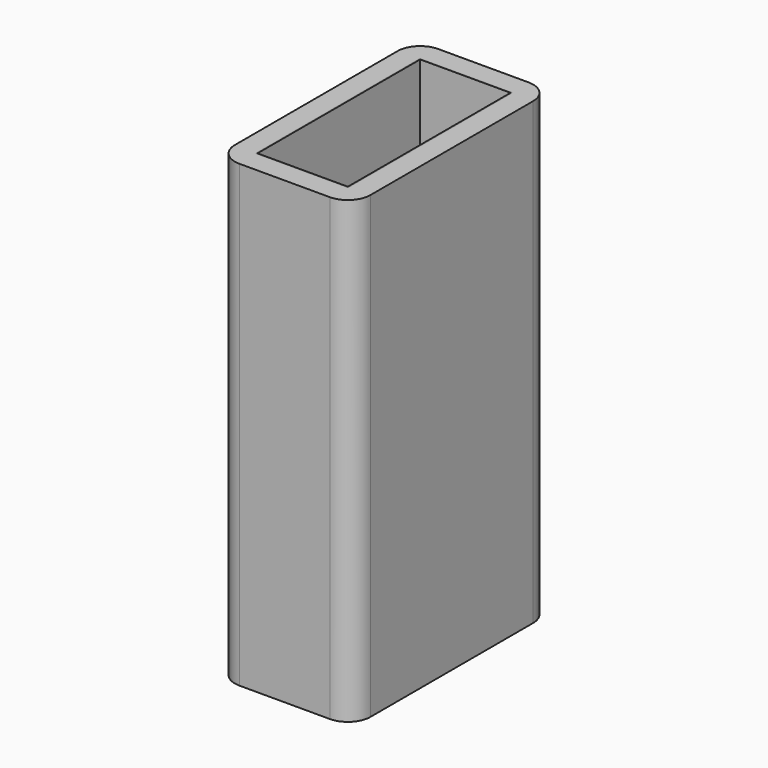
from build123d import *

# Parameters (mm, degrees)
F5_W      = 91.44
F5_H      = 167.64
F6_DEPTH  = 309.88
F7_R      = 15.24
F8_W      = 62.484
F8_H      = 138.684
F9_DEPTH  = 309.88
F10_W     = 62.484
F10_H     = 138.684
F11_DEPTH = 309.88
F12_W     = 60.96
F12_H     = 137.16
F13_DEPTH = 309.88
F14_R     = 0.762
F15_R     = 0.762


with BuildPart() as f6:
    # F5 (on Top) → F6 (new body)
    with BuildSketch(Plane.XY):
        Rectangle(F5_W, F5_H)
    extrude(amount=-F6_DEPTH)

    # F7
    f7_edges = [f6.edges().sort_by_distance(p)[0] for p in [
        (-45.72, 83.82, -154.94),
        (45.72, 83.82, -154.94),
        (45.72, -83.82, -154.94),
        (-45.72, -83.82, -154.94),
    ]]
    fillet(f7_edges, radius=F7_R)

    # F8 (on face) → F9 (cut)
    with BuildSketch(Plane.XY):
        Rectangle(F8_W, F8_H)
    extrude(amount=-F9_DEPTH, mode=Mode.SUBTRACT)

    # F15
    f15_edges = [f6.edges().sort_by_distance(p)[0] for p in [
        (-31.242, 69.342, -154.94),
        (-31.242, -69.342, -154.94),
        (31.242, -69.342, -154.94),
        (31.242, 69.342, -154.94),
    ]]
    fillet(f15_edges, radius=F15_R)


with BuildPart() as f11:
    # F10 (on face) → F11 (new body)
    with BuildSketch(Plane.XY):
        Rectangle(F10_W, F10_H)
    extrude(amount=-F11_DEPTH)

    # F12 (on face) → F13 (cut)
    with BuildSketch(Plane.XY):
        Rectangle(F12_W, F12_H)
    extrude(amount=-F13_DEPTH, mode=Mode.SUBTRACT)

    # F14
    f14_edges = [f11.edges().sort_by_distance(p)[0] for p in [
        (-31.242, 69.342, -154.94),
        (31.242, 69.342, -154.94),
        (31.242, -69.342, -154.94),
        (-31.242, -69.342, -154.94),
    ]]
    fillet(f14_edges, radius=F14_R)


solid = Compound([f6.part, f11.part])
